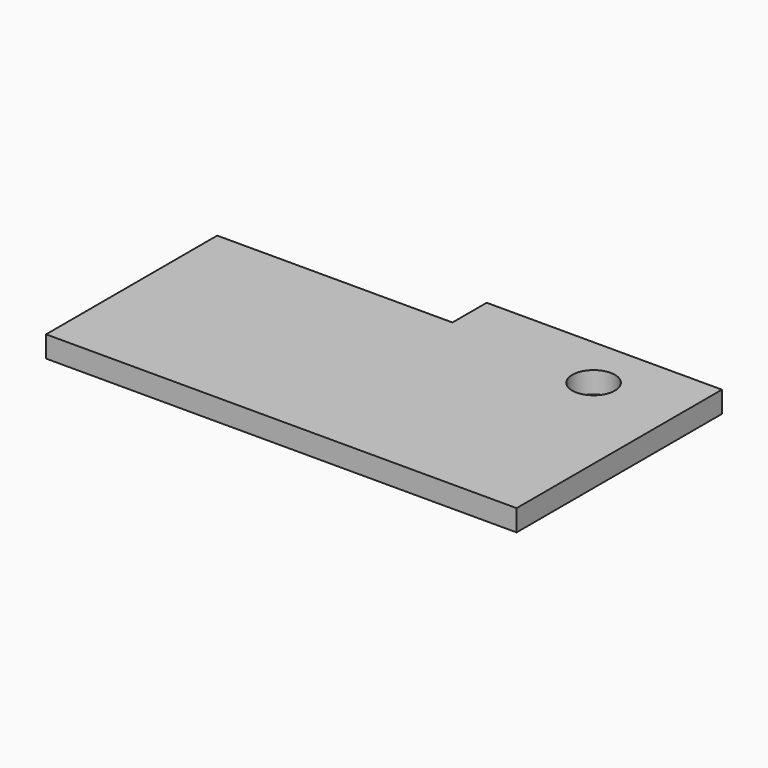
from build123d import *

# Parameters (mm, degrees)
F0_W     = 139.7
F0_H     = 25.4
F1_DEPTH = 12.7
F2_R     = 12.7
F3_DEPTH = 12.701


# Not quite as in the source:
# - a feature names something its author has since deleted; it is built from what else it names


with BuildPart() as f1:
    # F0 (on Top) → F1 (new body)
    with BuildSketch(Plane.XY):
        Polygon((0, 127), (0, 0), (279.4, 0), (279.4, 127), (139.7, 127), align=None)
        with Locations((209.55, 139.7)):
            Rectangle(F0_W, F0_H)
    extrude(amount=F1_DEPTH)

    # F2 (on face) → F3 (cut, through all)
    with BuildSketch(Plane.XY.offset(12.7)):
        with Locations((228.6, 120.65)):
            Circle(F2_R)
    extrude(amount=-F3_DEPTH, mode=Mode.SUBTRACT)


solid = f1.part
